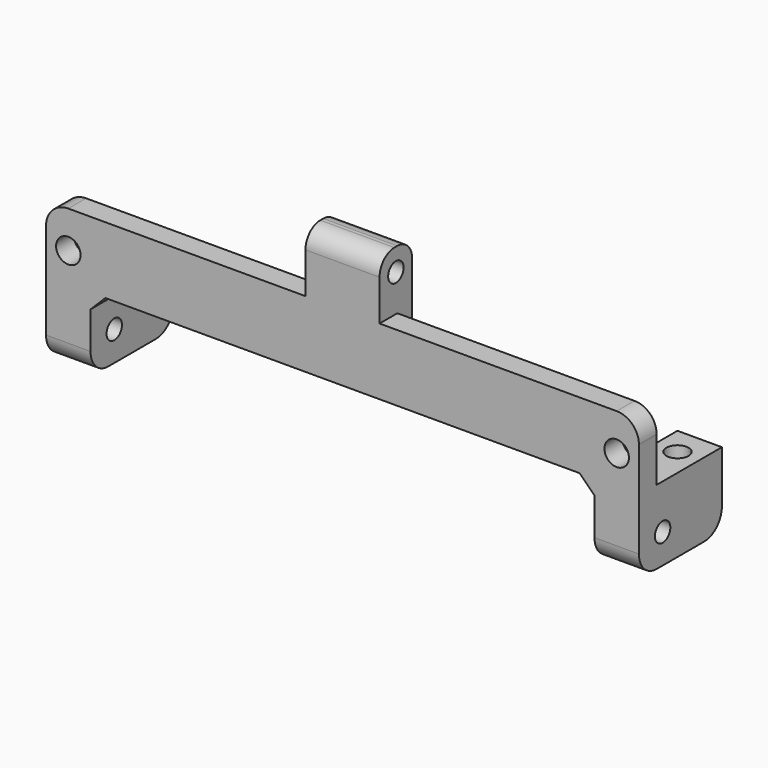
from build123d import *

# Parameters (mm, degrees)
F0_R      = 1.65
F1_DEPTH  = 14
F2_W      = 11
F2_H      = 9
F3_DEPTH  = 80.001
F4_R      = 1.3
F5_DEPTH  = 80.001
F6_R      = 3
F7_SIZE   = 2
F8_R      = 1.5
F9_DEPTH  = 3
F11_DEPTH = 2.5
F12_W     = 10
F12_H     = 8
F12_H_2   = 2
F13_DEPTH = 5.5
F14_R     = 2.5
F15_R     = 1.3
F16_DEPTH = 45.001


with BuildPart() as f1:
    # F0 (on Front) → F1 (new body)
    with BuildSketch(Plane.XZ):
        Polygon((-34, -4.5), (34, -4.5), (34, -14.5), (40, -14.5), (40, -4.5), (40, 4.5), (-40, 4.5), (-40, -4.5), (-40, -14.5), (-34, -14.5), align=None)
        with Locations((-37, -0.5)):
            Circle(F0_R, mode=Mode.SUBTRACT)
        with Locations((37, -0.5)):
            Circle(F0_R, mode=Mode.SUBTRACT)
    extrude(amount=F1_DEPTH)

    # F2 (on face) → F3 (cut, through all)
    with BuildSketch(Plane.YZ.offset(40)):
        with Locations((-5.5, 0)):
            Rectangle(F2_W, F2_H)
    extrude(amount=-F3_DEPTH, mode=Mode.SUBTRACT)

    # F4 (on face) → F5 (cut, through all)
    with BuildSketch(Plane.YZ.offset(40)):
        with Locations((-10, -10.5)):
            Circle(F4_R)
    extrude(amount=-F5_DEPTH, mode=Mode.SUBTRACT)

    # F6
    f6_edges = [f1.edges().sort_by_distance(p)[0] for p in [
        (37, -14, -14.5),
        (-37, -14, -14.5),
        (-37, 0, -14.5),
        (37, 0, -14.5),
        (40, -12.5, 4.5),
        (-40, -12.5, 4.5),
    ]]
    fillet(f6_edges, radius=F6_R)

    # F7
    f7_edges = [f1.edges().sort_by_distance(p)[0] for p in [
        (34, -12.5, -4.5),
        (-34, -12.5, -4.5),
    ]]
    chamfer(f7_edges, length=F7_SIZE)

    # F8 (on face) → F9 (cut)
    with BuildSketch(Plane.XY.offset(-4.5)):
        with Locations((-37, -3.75)):
            Circle(F8_R)
        with Locations((37, -3.75)):
            Circle(F8_R)
    extrude(amount=-F9_DEPTH, mode=Mode.SUBTRACT)

    # F10 (on face) → F11 (join)
    with BuildSketch(Plane(origin=(0, -11, 0), x_dir=(-1, 0, 0), z_dir=(0, 1, 0))):
        Polygon((-5, 2.5), (-30, 2.5), (-30, -4.5), (30, -4.5), (30, 2.5), (5, 2.5), (5, 4.5), (-5, 4.5), align=None)
    extrude(amount=F11_DEPTH)

    # F12 (on face) → F13 (join)
    with BuildSketch(Plane(origin=(0, -8.5, 0), x_dir=(-1, 0, 0), z_dir=(0, 1, 0))):
        with Locations((0, 8.5)):
            Rectangle(F12_W, F12_H)
        with Locations((0, 3.5)):
            Rectangle(F12_W, F12_H_2)
    extrude(amount=-F13_DEPTH)

    # F14
    f14_edges = [f1.edges().sort_by_distance(p)[0] for p in [
        (0, -14, 12.5),
        (0, -8.5, 12.5),
    ]]
    fillet(f14_edges, radius=F14_R)

    # F15 (on face) → F16 (cut, through all)
    with BuildSketch(Plane.YZ.offset(5)):
        with Locations((-11.25, 9.5)):
            Circle(F15_R)
    extrude(amount=-F16_DEPTH, mode=Mode.SUBTRACT)


solid = f1.part
